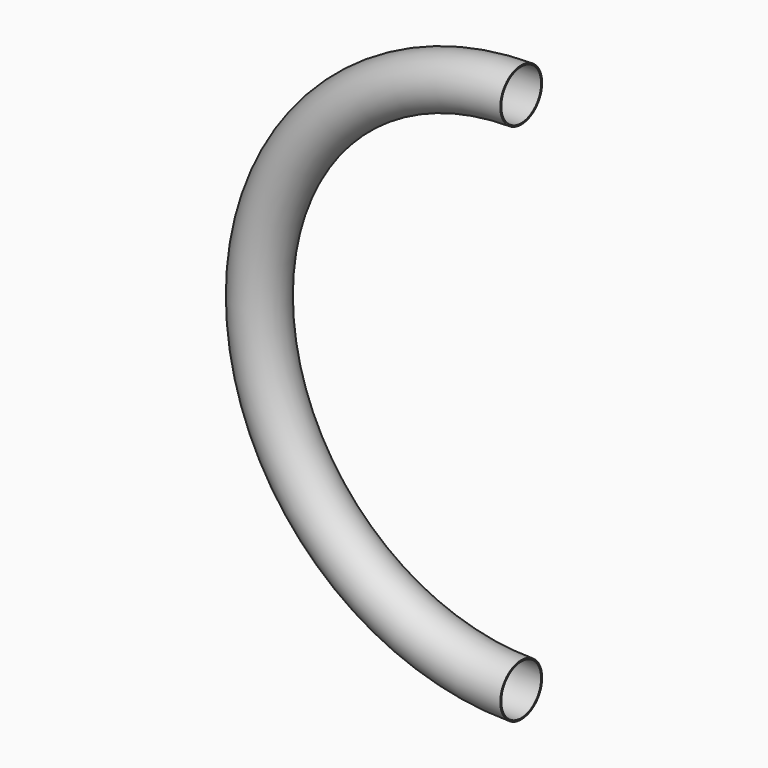
from build123d import *

# Parameters (mm, degrees)
F0_R   = 10
F0_R_2 = 9.5


with BuildPart() as f2:
    # F2: sweep along a path in F1
    with BuildLine(Plane.XZ) as f2_path:
        ThreePointArc((0, 200), (-100, 100), (0, 0))
    # F0 (on Right) → F2 (sweep)
    with BuildSketch(Plane.YZ):
        Circle(F0_R)
        Circle(F0_R_2, mode=Mode.SUBTRACT)
    sweep(path=f2_path.line)


solid = f2.part
